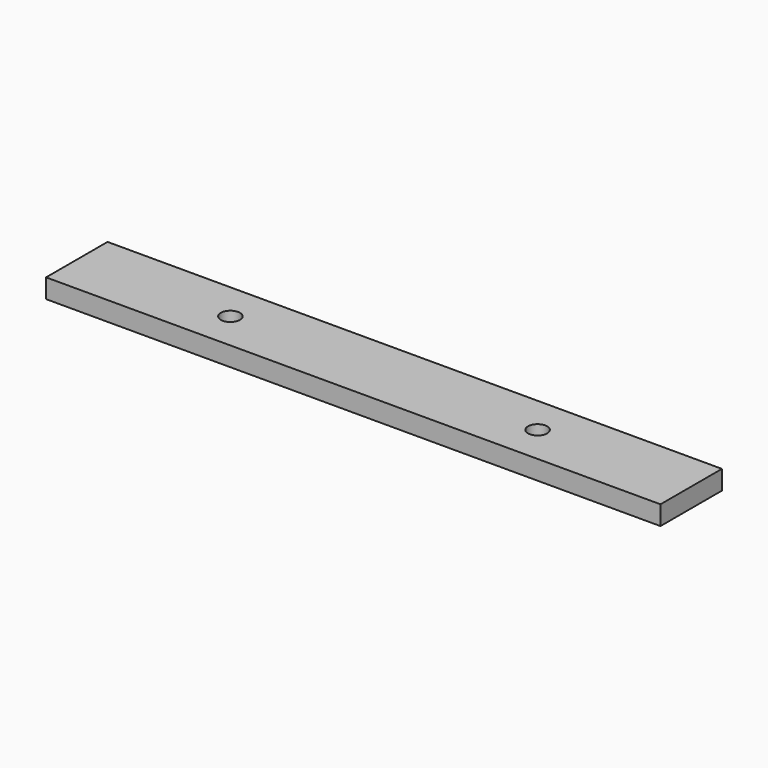
from build123d import *

# Parameters (mm, degrees)
F0_R     = 3.175
F1_DEPTH = 6.35


# Not quite as in the source:
# - a feature names something its author has since deleted; it is built from what else it names


with BuildPart() as f1:
    # F0 (on Top) → F1 (new body)
    with BuildSketch(Plane.XY):
        Polygon((88.9, -116.7384), (76.2, -116.7384), (-76.2, -116.7384), (-101.6, -116.7384), (-101.6, -142.1384), (101.6, -142.1384), (101.6, -116.7384), align=None)
        with Locations((-50.8, -129.4384)):
            Circle(F0_R, mode=Mode.SUBTRACT)
        with Locations((50.8, -129.4384)):
            Circle(F0_R, mode=Mode.SUBTRACT)
    extrude(amount=F1_DEPTH)


solid = f1.part
